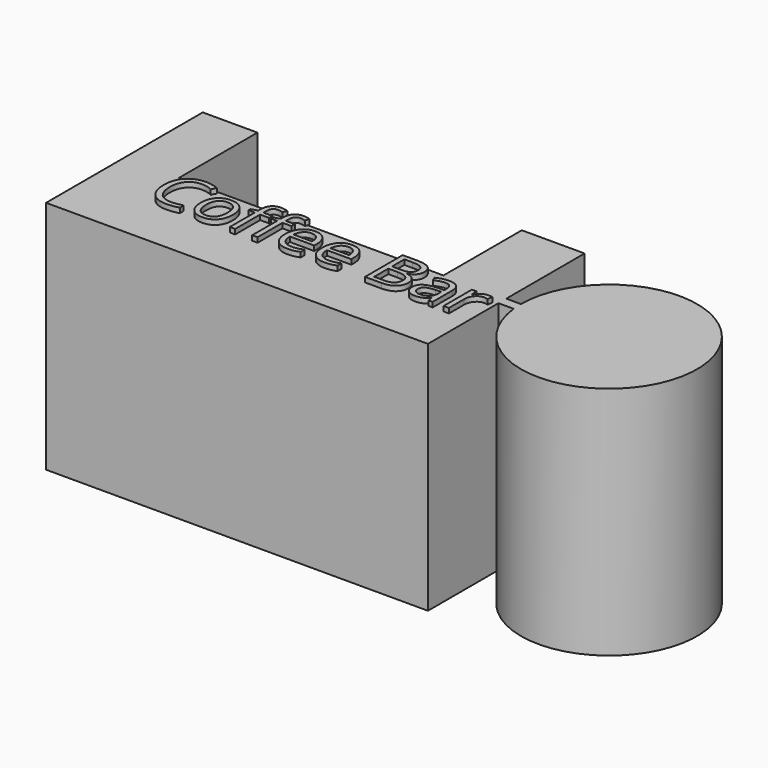
from build123d import *

# Parameters (mm, degrees)
F1_DEPTH     = 1219.2
F2_TEXT_SIZE = 342.3669055803
F3_DEPTH     = 25.4
F4_R         = 457.2
F5_DEPTH     = 1016
F5_TAPER     = 12


# Not quite as in the source:
# - Text() gives the source's letters only with a copy of the font that has no kerning and outlines rounded to 1/6400 em; it was checked with that copy


with BuildPart() as f1:
    # F0 (on Top) → F1 (new body)
    with BuildSketch(Plane.XY):
        with BuildLine():
            Line((-990.6, -508), (990.6, -508))
            Line((990.6, -508), (990.6, -50.8))
            Line((990.6, -50.8), (1069.630986972, -50.8))
            ThreePointArc((1069.630986972, -50.8), (1980.4917046105, 25.4394107992), (1066.8, 0))
            Line((1066.8, 0), (990.6, 0))
            Line((990.6, 0), (990.6, 508))
            Line((990.6, 508), (664.8090759277, 508))
            Line((664.8090759277, 508), (664.8090759277, 0))
            Line((664.8090759277, 0), (-706.7909240723, 0))
            Line((-706.7909240723, 0), (-706.7909240723, 508))
            Line((-706.7909240723, 508), (-990.6, 508))
            Line((-990.6, 508), (-990.6, -508))
        make_face()
    extrude(amount=-F1_DEPTH)

    # F2 (on face) → F3 (join)
    with BuildSketch(Plane.XY):
        with Locations((-706.7909240723, -246.5041720178)):
            Text('Coffee Bar', F2_TEXT_SIZE, font='Open Sans', text_align=(TextAlign.LEFT, TextAlign.BOTTOM))
    extrude(amount=F3_DEPTH)


with BuildPart() as f5:
    # F4 (on face) → F5 (new body)
    with BuildSketch(Plane.XY):
        with Locations((1414.8636444476, 0)):
            Circle(F4_R)
    extrude(amount=-F5_DEPTH, taper=F5_TAPER)


solid = f1.part
